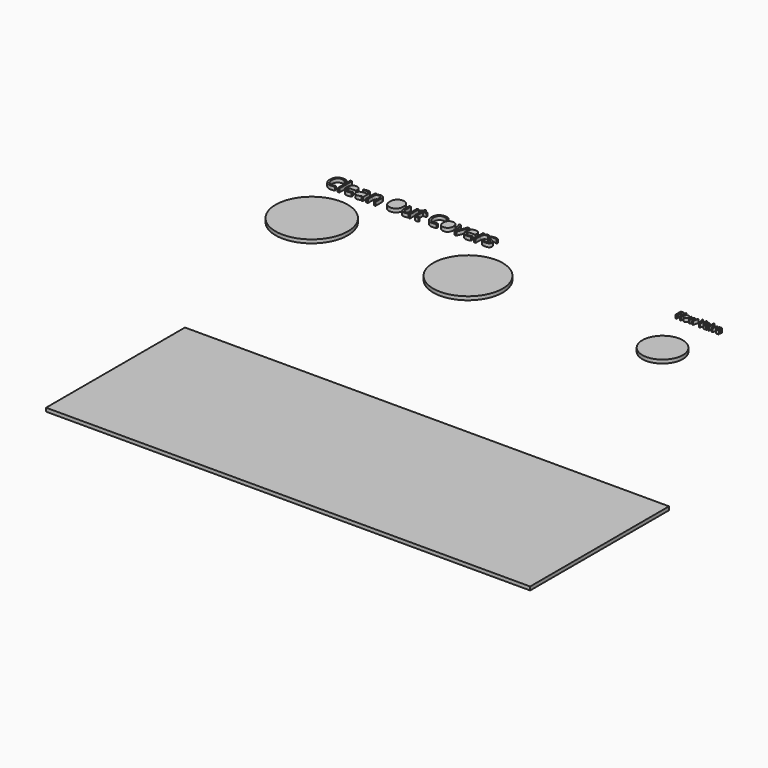
from build123d import *

# Parameters (mm, degrees)
F0_W           = 4170.580181663
F0_H           = 1495.7776816476
F0_W_2         = 38.067660993
F0_H_2         = 356.6917830613
F0_H_3         = 251.2172233158
F0_R           = 311.3295690079
F0_R_2         = 299.2849043025
F0_R_3         = 174.2052882787
F0_TEXT_SIZE   = 179.4427633286
F0_TEXT_SIZE_2 = 469.4278041522
F0_TEXT_SIZE_3 = 78.9547959963
F1_DEPTH       = 30.48


# Not quite as in the source:
# - Text() gives the source's letters only with a copy of the font that has no kerning and outlines rounded to 1/6400 em; it was checked with that copy


with BuildPart() as f1:
    # F0 (on Top) → F1 (new body)
    with BuildSketch(Plane.XY):
        with Locations((453.2191234097, -1260.6751158237)):
            Rectangle(F0_W, F0_H)
        with BuildLine():
            add(Edge.make_bspline(
                [(-404.8579966184, -1421.0070061187), (-364.2965004159, -1466.8495651179), (-364.2965004159, -1547.5324689566)],
                knots=[0, 0, 0, 1, 1, 1], degree=2))
            add(Edge.make_bspline(
                [(-364.2965004159, -1547.5324689566), (-364.2965004159, -1627.995328512), (-405.0046928072, -1674.0946058417)],
                knots=[0, 0, 0, 1, 1, 1], degree=2))
            add(Edge.make_bspline(
                [(-405.0046928072, -1674.0946058417), (-445.7128851985, -1720.1938831713), (-518.1074543701, -1720.1938831713)],
                knots=[0, 0, 0, 1, 1, 1], degree=2))
            add(Edge.make_bspline(
                [(-518.1074543701, -1720.1938831713), (-592.1156816185, -1720.1938831713), (-632.3471113962, -1674.9014348801)],
                knots=[0, 0, 0, 1, 1, 1], degree=2))
            add(Edge.make_bspline(
                [(-632.3471113962, -1674.9014348801), (-672.5785411739, -1629.6089865888), (-672.5785411739, -1547.0923803902)],
                knots=[0, 0, 0, 1, 1, 1], degree=2))
            add(Edge.make_bspline(
                [(-672.5785411739, -1547.0923803902), (-672.5785411739, -1465.2359070412), (-632.2370892546, -1420.2001770803)],
                knots=[0, 0, 0, 1, 1, 1], degree=2))
            add(Edge.make_bspline(
                [(-632.2370892546, -1420.2001770803), (-591.8956373353, -1375.1644471195), (-517.6673658037, -1375.1644471195)],
                knots=[0, 0, 0, 1, 1, 1], degree=2))
            add(Edge.make_bspline(
                [(-517.6673658037, -1375.1644471195), (-445.4194928209, -1375.1644471195), (-404.8579966184, -1421.0070061187)],
                knots=[0, 0, 0, 1, 1, 1], degree=2))
        make_face(mode=Mode.SUBTRACT)
        with Locations((-276.3154611845, -1537.2270616936)):
            Rectangle(F0_W_2, F0_H_2, mode=Mode.SUBTRACT)
        with BuildLine():
            Line((-0.5633002923, -1715.5729532242), (-5.6243188058, -1681.9061778951))
            Line((-5.6243188058, -1681.9061778951), (-7.678065449, -1681.9061778951))
            add(Edge.make_bspline(
                [(-7.678065449, -1681.9061778951), (-34.0100313382, -1720.1938831713), (-86.5272669277, -1720.1938831713)],
                knots=[0, 0, 0, 1, 1, 1], degree=2))
            add(Edge.make_bspline(
                [(-86.5272669277, -1720.1938831713), (-135.8171863637, -1720.1938831713), (-163.2126996216, -1686.4904337951)],
                knots=[0, 0, 0, 1, 1, 1], degree=2))
            add(Edge.make_bspline(
                [(-163.2126996216, -1686.4904337951), (-190.6082128795, -1652.7869844188), (-190.6082128795, -1590.6611484631)],
                knots=[0, 0, 0, 1, 1, 1], degree=2))
            add(Edge.make_bspline(
                [(-190.6082128795, -1590.6611484631), (-190.6082128795, -1528.5353125073), (-163.10267748, -1494.1350562343)],
                knots=[0, 0, 0, 1, 1, 1], degree=2))
            add(Edge.make_bspline(
                [(-163.10267748, -1494.1350562343), (-135.5971420805, -1459.7347999612), (-86.5272669277, -1459.7347999612)],
                knots=[0, 0, 0, 1, 1, 1], degree=2))
            add(Edge.make_bspline(
                [(-86.5272669277, -1459.7347999612), (-35.4036451317, -1459.7347999612), (-8.1181540154, -1496.9222838214)],
                knots=[0, 0, 0, 1, 1, 1], degree=2))
            Line((-8.1181540154, -1496.9222838214), (-5.110882145, -1496.9222838214))
            Line((-5.110882145, -1496.9222838214), (-6.7245402218, -1478.8053045049))
            Line((-6.7245402218, -1478.8053045049), (-7.678065449, -1461.1284137548))
            Line((-7.678065449, -1461.1284137548), (-7.678065449, -1358.8811701629))
            Line((-7.678065449, -1358.8811701629), (30.389595544, -1358.8811701629))
            Line((30.389595544, -1358.8811701629), (30.389595544, -1715.5729532242))
            Line((30.389595544, -1715.5729532242), (-0.5633002923, -1715.5729532242))
        make_face(mode=Mode.SUBTRACT)
        with BuildLine():
            add(Edge.make_bspline(
                [(325.6890235934, -1380.4455099162), (451.2609612041, -1380.4455099162), (451.2609612041, -1478.0718235609)],
                knots=[0, 0, 0, 1, 1, 1], degree=2))
            add(Edge.make_bspline(
                [(451.2609612041, -1478.0718235609), (451.2609612041, -1528.9754010737), (416.5306385063, -1556.3709143316)],
                knots=[0, 0, 0, 1, 1, 1], degree=2))
            add(Edge.make_bspline(
                [(416.5306385063, -1556.3709143316), (381.8003158085, -1583.7664275896), (317.1806446432, -1583.7664275896)],
                knots=[0, 0, 0, 1, 1, 1], degree=2))
            Line((317.1806446432, -1583.7664275896), (277.7193698566, -1583.7664275896))
            Line((277.7193698566, -1583.7664275896), (277.7193698566, -1715.5729532242))
            Line((277.7193698566, -1715.5729532242), (238.7715317309, -1715.5729532242))
            Line((238.7715317309, -1715.5729532242), (238.7715317309, -1380.4455099162))
            Line((238.7715317309, -1380.4455099162), (325.6890235934, -1380.4455099162))
        make_face(mode=Mode.SUBTRACT)
        with BuildLine():
            Line((698.3706912336, -1715.5729532242), (670.1316748901, -1715.5729532242))
            Line((670.1316748901, -1715.5729532242), (662.576821167, -1679.7790831576))
            Line((662.576821167, -1679.7790831576), (660.7431188071, -1679.7790831576))
            add(Edge.make_bspline(
                [(660.7431188071, -1679.7790831576), (641.966006641, -1703.397169554), (623.2989166165, -1711.7955263626)],
                knots=[0, 0, 0, 1, 1, 1], degree=2))
            add(Edge.make_bspline(
                [(623.2989166165, -1711.7955263626), (604.631826592, -1720.1938831713), (576.6128545317, -1720.1938831713)],
                knots=[0, 0, 0, 1, 1, 1], degree=2))
            add(Edge.make_bspline(
                [(576.6128545317, -1720.1938831713), (539.2786744827, -1720.1938831713), (518.0810752014, -1700.9033343444)],
                knots=[0, 0, 0, 1, 1, 1], degree=2))
            add(Edge.make_bspline(
                [(518.0810752014, -1700.9033343444), (496.8834759202, -1681.6127855175), (496.8834759202, -1646.1123078285)],
                knots=[0, 0, 0, 1, 1, 1], degree=2))
            add(Edge.make_bspline(
                [(496.8834759202, -1646.1123078285), (496.8834759202, -1570.050333937), (618.5679645278, -1566.3829292171)],
                knots=[0, 0, 0, 1, 1, 1], degree=2))
            Line((618.5679645278, -1566.3829292171), (661.1832073734, -1564.9893154235))
            Line((661.1832073734, -1564.9893154235), (661.1832073734, -1549.3661713166))
            add(Edge.make_bspline(
                [(661.1832073734, -1549.3661713166), (661.1832073734, -1519.8068892738), (648.4939870425, -1505.7240551493)],
                knots=[0, 0, 0, 1, 1, 1], degree=2))
            add(Edge.make_bspline(
                [(648.4939870425, -1505.7240551493), (635.8047667115, -1491.6412210247), (607.7857946511, -1491.6412210247)],
                knots=[0, 0, 0, 1, 1, 1], degree=2))
            add(Edge.make_bspline(
                [(607.7857946511, -1491.6412210247), (576.3928102485, -1491.6412210247), (536.7848392731, -1510.8584217572)],
                knots=[0, 0, 0, 1, 1, 1], degree=2))
            Line((536.7848392731, -1510.8584217572), (525.0491441693, -1481.7392282809))
            add(Edge.make_bspline(
                [(525.0491441693, -1481.7392282809), (543.6062120522, -1471.6905393482), (565.7206625134, -1465.9693879851)],
                knots=[0, 0, 0, 1, 1, 1], degree=2))
            add(Edge.make_bspline(
                [(565.7206625134, -1465.9693879851), (587.8351129747, -1460.248236622), (610.1329336719, -1460.248236622)],
                knots=[0, 0, 0, 1, 1, 1], degree=2))
            add(Edge.make_bspline(
                [(610.1329336719, -1460.248236622), (655.0219674439, -1460.248236622), (676.6963293388, -1480.1622442513)],
                knots=[0, 0, 0, 1, 1, 1], degree=2))
            add(Edge.make_bspline(
                [(676.6963293388, -1480.1622442513), (698.3706912336, -1500.0762518806), (698.3706912336, -1544.0851085198)],
                knots=[0, 0, 0, 1, 1, 1], degree=2))
            Line((698.3706912336, -1544.0851085198), (698.3706912336, -1715.5729532242))
        make_face(mode=Mode.SUBTRACT)
        with BuildLine():
            add(Edge.make_bspline(
                [(828.2701664139, -1676.5884410512), (839.0523362905, -1688.7275506742), (857.8294484566, -1688.7275506742)],
                knots=[0, 0, 0, 1, 1, 1], degree=2))
            add(Edge.make_bspline(
                [(857.8294484566, -1688.7275506742), (867.9514854836, -1688.7275506742), (877.3400415666, -1687.2605887863)],
                knots=[0, 0, 0, 1, 1, 1], degree=2))
            add(Edge.make_bspline(
                [(877.3400415666, -1687.2605887863), (886.7285976497, -1685.7936268983), (892.2297047296, -1684.1799688215)],
                knots=[0, 0, 0, 1, 1, 1], degree=2))
            Line((892.2297047296, -1684.1799688215), (892.2297047296, -1713.2991622978))
            add(Edge.make_bspline(
                [(892.2297047296, -1713.2991622978), (886.0684648001, -1716.2330860738), (874.0393773187, -1718.2134846225)],
                knots=[0, 0, 0, 1, 1, 1], degree=2))
            add(Edge.make_bspline(
                [(874.0393773187, -1718.2134846225), (862.0102898373, -1720.1938831713), (852.3283413767, -1720.1938831713)],
                knots=[0, 0, 0, 1, 1, 1], degree=2))
            add(Edge.make_bspline(
                [(852.3283413767, -1720.1938831713), (779.4936836387, -1720.1938831713), (779.4936836387, -1643.3984283358)],
                knots=[0, 0, 0, 1, 1, 1], degree=2))
            Line((779.4936836387, -1643.3984283358), (779.4936836387, -1493.9150119511))
            Line((779.4936836387, -1493.9150119511), (743.4797692889, -1493.9150119511))
            Line((743.4797692889, -1493.9150119511), (743.4797692889, -1475.5779883514))
            Line((743.4797692889, -1475.5779883514), (779.4936836387, -1459.7347999612))
            Line((779.4936836387, -1459.7347999612), (795.4835682176, -1406.1173429557))
            Line((795.4835682176, -1406.1173429557), (817.4879965372, -1406.1173429557))
            Line((817.4879965372, -1406.1173429557), (817.4879965372, -1464.3557299084))
            Line((817.4879965372, -1464.3557299084), (890.3960023696, -1464.3557299084))
            Line((890.3960023696, -1464.3557299084), (890.3960023696, -1493.9150119511))
            Line((890.3960023696, -1493.9150119511), (817.4879965372, -1493.9150119511))
            Line((817.4879965372, -1493.9150119511), (817.4879965372, -1641.784770259))
            add(Edge.make_bspline(
                [(817.4879965372, -1641.784770259), (817.4879965372, -1664.4493314282), (828.2701664139, -1676.5884410512)],
                knots=[0, 0, 0, 1, 1, 1], degree=2))
        make_face(mode=Mode.SUBTRACT)
        with Locations((961.4336317948, -1589.9643415663)):
            Rectangle(F0_W_2, F0_H_3, mode=Mode.SUBTRACT)
        with BuildLine():
            add(Edge.make_bspline(
                [(1246.9044151949, -1494.8318631311), (1277.9673331728, -1529.9289263009), (1277.9673331728, -1589.7076232359)],
                knots=[0, 0, 0, 1, 1, 1], degree=2))
            add(Edge.make_bspline(
                [(1277.9673331728, -1589.7076232359), (1277.9673331728, -1651.1733263421), (1247.0511113837, -1685.6836047567)],
                knots=[0, 0, 0, 1, 1, 1], degree=2))
            add(Edge.make_bspline(
                [(1247.0511113837, -1685.6836047567), (1216.1348895946, -1720.1938831713), (1161.5639073619, -1720.1938831713)],
                knots=[0, 0, 0, 1, 1, 1], degree=2))
            add(Edge.make_bspline(
                [(1161.5639073619, -1720.1938831713), (1127.8237839385, -1720.1938831713), (1101.7118623325, -1704.3506947812)],
                knots=[0, 0, 0, 1, 1, 1], degree=2))
            add(Edge.make_bspline(
                [(1101.7118623325, -1704.3506947812), (1075.5999407265, -1688.507506391), (1061.3704104132, -1658.9482243483)],
                knots=[0, 0, 0, 1, 1, 1], degree=2))
            add(Edge.make_bspline(
                [(1061.3704104132, -1658.9482243483), (1047.1408800998, -1629.3889423056), (1047.1408800998, -1589.7076232359)],
                knots=[0, 0, 0, 1, 1, 1], degree=2))
            add(Edge.make_bspline(
                [(1047.1408800998, -1589.7076232359), (1047.1408800998, -1528.3152682241), (1077.8737316529, -1494.0250340927)],
                knots=[0, 0, 0, 1, 1, 1], degree=2))
            add(Edge.make_bspline(
                [(1077.8737316529, -1494.0250340927), (1108.606583206, -1459.7347999612), (1163.1775654387, -1459.7347999612)],
                knots=[0, 0, 0, 1, 1, 1], degree=2))
            add(Edge.make_bspline(
                [(1163.1775654387, -1459.7347999612), (1215.841497217, -1459.7347999612), (1246.9044151949, -1494.8318631311)],
                knots=[0, 0, 0, 1, 1, 1], degree=2))
        make_face(mode=Mode.SUBTRACT)
        with BuildLine():
            add(Edge.make_bspline(
                [(945.5904434047, -1415.4325509444), (939.1724851448, -1409.1246148261), (939.1724851448, -1396.2886983063)],
                knots=[0, 0, 0, 1, 1, 1], degree=2))
            add(Edge.make_bspline(
                [(939.1724851448, -1396.2886983063), (939.1724851448, -1383.2327375033), (945.5904434047, -1377.1448456682)],
                knots=[0, 0, 0, 1, 1, 1], degree=2))
            add(Edge.make_bspline(
                [(945.5904434047, -1377.1448456682), (952.0084016646, -1371.0569538331), (961.6903501252, -1371.0569538331)],
                knots=[0, 0, 0, 1, 1, 1], degree=2))
            add(Edge.make_bspline(
                [(961.6903501252, -1371.0569538331), (970.8588619251, -1371.0569538331), (977.4968644682, -1377.2548678098)],
                knots=[0, 0, 0, 1, 1, 1], degree=2))
            add(Edge.make_bspline(
                [(977.4968644682, -1377.2548678098), (984.1348670113, -1383.4527817865), (984.1348670113, -1396.2886983063)],
                knots=[0, 0, 0, 1, 1, 1], degree=2))
            add(Edge.make_bspline(
                [(984.1348670113, -1396.2886983063), (984.1348670113, -1409.1246148261), (977.4968644682, -1415.4325509444)],
                knots=[0, 0, 0, 1, 1, 1], degree=2))
            add(Edge.make_bspline(
                [(977.4968644682, -1415.4325509444), (970.8588619251, -1421.7404870627), (961.6903501252, -1421.7404870627)],
                knots=[0, 0, 0, 1, 1, 1], degree=2))
            add(Edge.make_bspline(
                [(961.6903501252, -1421.7404870627), (952.0084016646, -1421.7404870627), (945.5904434047, -1415.4325509444)],
                knots=[0, 0, 0, 1, 1, 1], degree=2))
        make_face(mode=Mode.SUBTRACT)
        with Locations((-1962.2709674218, 1265.2137250001)):
            Circle(F0_R)
        with Locations((-616.0709674218, 1265.2137250001)):
            Circle(F0_R_2)
        with Locations((1060.3290325782, 1265.2137250001)):
            Circle(F0_R_3)
        with BuildLine():
            add(Edge.make_bspline(
                [(-602.3477407871, -1445.2118772703), (-631.3569121218, -1480.4189625817), (-631.3569121218, -1547.5324689566)],
                knots=[0, 0, 0, 1, 1, 1], degree=2))
            add(Edge.make_bspline(
                [(-631.3569121218, -1547.5324689566), (-631.3569121218, -1615.5995005586), (-602.3477407871, -1650.8065858701)],
                knots=[0, 0, 0, 1, 1, 1], degree=2))
            add(Edge.make_bspline(
                [(-602.3477407871, -1650.8065858701), (-573.3385694524, -1686.0136711815), (-518.1074543701, -1686.0136711815)],
                knots=[0, 0, 0, 1, 1, 1], degree=2))
            add(Edge.make_bspline(
                [(-518.1074543701, -1686.0136711815), (-462.4362507214, -1686.0136711815), (-434.0138641419, -1650.9532820589)],
                knots=[0, 0, 0, 1, 1, 1], degree=2))
            add(Edge.make_bspline(
                [(-434.0138641419, -1650.9532820589), (-405.5914775624, -1615.8928929362), (-405.5914775624, -1547.5324689566)],
                knots=[0, 0, 0, 1, 1, 1], degree=2))
            add(Edge.make_bspline(
                [(-405.5914775624, -1547.5324689566), (-405.5914775624, -1479.9055259209), (-433.9038420003, -1444.9551589399)],
                knots=[0, 0, 0, 1, 1, 1], degree=2))
            add(Edge.make_bspline(
                [(-433.9038420003, -1444.9551589399), (-462.2162064382, -1410.0047919589), (-517.6673658037, -1410.0047919589)],
                knots=[0, 0, 0, 1, 1, 1], degree=2))
            add(Edge.make_bspline(
                [(-517.6673658037, -1410.0047919589), (-573.3385694524, -1410.0047919589), (-602.3477407871, -1445.2118772703)],
                knots=[0, 0, 0, 1, 1, 1], degree=2))
        make_face()
        with BuildLine():
            add(Edge.make_bspline(
                [(1105.6359853828, -1516.6162471675), (1086.6021548863, -1541.1511847439), (1086.6021548863, -1589.7076232359)],
                knots=[0, 0, 0, 1, 1, 1], degree=2))
            add(Edge.make_bspline(
                [(1086.6021548863, -1589.7076232359), (1086.6021548863, -1637.8973212559), (1105.856029666, -1663.0923916819)],
                knots=[0, 0, 0, 1, 1, 1], degree=2))
            add(Edge.make_bspline(
                [(1105.856029666, -1663.0923916819), (1125.1099044457, -1688.2874621078), (1162.4440844947, -1688.2874621078)],
                knots=[0, 0, 0, 1, 1, 1], degree=2))
            add(Edge.make_bspline(
                [(1162.4440844947, -1688.2874621078), (1199.8516126381, -1688.2874621078), (1219.2155095593, -1663.2024138235)],
                knots=[0, 0, 0, 1, 1, 1], degree=2))
            add(Edge.make_bspline(
                [(1219.2155095593, -1663.2024138235), (1238.5794064806, -1638.1173655391), (1238.5794064806, -1589.7076232359)],
                knots=[0, 0, 0, 1, 1, 1], degree=2))
            add(Edge.make_bspline(
                [(1238.5794064806, -1589.7076232359), (1238.5794064806, -1541.8113175935), (1219.2155095593, -1516.9463135923)],
                knots=[0, 0, 0, 1, 1, 1], degree=2))
            add(Edge.make_bspline(
                [(1219.2155095593, -1516.9463135923), (1199.8516126381, -1492.0813095911), (1162.0039959283, -1492.0813095911)],
                knots=[0, 0, 0, 1, 1, 1], degree=2))
            add(Edge.make_bspline(
                [(1162.0039959283, -1492.0813095911), (1124.6698158793, -1492.0813095911), (1105.6359853828, -1516.6162471675)],
                knots=[0, 0, 0, 1, 1, 1], degree=2))
        make_face()
        with BuildLine():
            add(Edge.make_bspline(
                [(-133.5067213901, -1663.7525245314), (-115.8665046872, -1688.2874621078), (-81.6862926974, -1688.2874621078)],
                knots=[0, 0, 0, 1, 1, 1], degree=2))
            add(Edge.make_bspline(
                [(-81.6862926974, -1688.2874621078), (-42.7384545716, -1688.2874621078), (-25.2082600103, -1667.0898628266)],
                knots=[0, 0, 0, 1, 1, 1], degree=2))
            add(Edge.make_bspline(
                [(-25.2082600103, -1667.0898628266), (-7.678065449, -1645.8922635453), (-7.678065449, -1598.6560907525)],
                knots=[0, 0, 0, 1, 1, 1], degree=2))
            Line((-7.678065449, -1598.6560907525), (-7.678065449, -1590.6611484631))
            add(Edge.make_bspline(
                [(-7.678065449, -1590.6611484631), (-7.678065449, -1537.2637357408), (-25.4283042935, -1514.4524783827)],
                knots=[0, 0, 0, 1, 1, 1], degree=2))
            add(Edge.make_bspline(
                [(-25.4283042935, -1514.4524783827), (-43.178543138, -1491.6412210247), (-82.1263812638, -1491.6412210247)],
                knots=[0, 0, 0, 1, 1, 1], degree=2))
            add(Edge.make_bspline(
                [(-82.1263812638, -1491.6412210247), (-115.646460404, -1491.6412210247), (-133.3966992485, -1517.6431204891)],
                knots=[0, 0, 0, 1, 1, 1], degree=2))
            add(Edge.make_bspline(
                [(-133.3966992485, -1517.6431204891), (-151.146938093, -1543.6450199534), (-151.146938093, -1591.1012370295)],
                knots=[0, 0, 0, 1, 1, 1], degree=2))
            add(Edge.make_bspline(
                [(-151.146938093, -1591.1012370295), (-151.146938093, -1639.2175869551), (-133.5067213901, -1663.7525245314)],
                knots=[0, 0, 0, 1, 1, 1], degree=2))
        make_face()
        with BuildLine():
            Line((277.7193698566, -1414.1856333396), (277.7193698566, -1550.3196965437))
            Line((277.7193698566, -1550.3196965437), (312.8531070737, -1550.3196965437))
            add(Edge.make_bspline(
                [(312.8531070737, -1550.3196965437), (364.6368617192, -1550.3196965437), (387.778185502, -1533.5963310208)],
                knots=[0, 0, 0, 1, 1, 1], degree=2))
            add(Edge.make_bspline(
                [(387.778185502, -1533.5963310208), (410.9195092848, -1516.8729654979), (410.9195092848, -1479.9055259209)],
                knots=[0, 0, 0, 1, 1, 1], degree=2))
            add(Edge.make_bspline(
                [(410.9195092848, -1479.9055259209), (410.9195092848, -1446.6788391583), (389.1351252484, -1430.4322362489)],
                knots=[0, 0, 0, 1, 1, 1], degree=2))
            add(Edge.make_bspline(
                [(389.1351252484, -1430.4322362489), (367.3507412119, -1414.1856333396), (321.2881379295, -1414.1856333396)],
                knots=[0, 0, 0, 1, 1, 1], degree=2))
            Line((321.2881379295, -1414.1856333396), (277.7193698566, -1414.1856333396))
        make_face()
        with BuildLine():
            add(Edge.make_bspline(
                [(549.2540153209, -1677.9820548448), (561.7231913687, -1688.7275506742), (584.1677082547, -1688.7275506742)],
                knots=[0, 0, 0, 1, 1, 1], degree=2))
            add(Edge.make_bspline(
                [(584.1677082547, -1688.7275506742), (619.7415340381, -1688.7275506742), (640.0222821394, -1669.2536316114)],
                knots=[0, 0, 0, 1, 1, 1], degree=2))
            add(Edge.make_bspline(
                [(640.0222821394, -1669.2536316114), (660.3030302407, -1649.7797125485), (660.3030302407, -1614.7193234259)],
                knots=[0, 0, 0, 1, 1, 1], degree=2))
            Line((660.3030302407, -1614.7193234259), (660.3030302407, -1592.0547622566))
            Line((660.3030302407, -1592.0547622566), (622.2353692477, -1593.595072239))
            add(Edge.make_bspline(
                [(622.2353692477, -1593.595072239), (576.8328988149, -1595.2087303158), (556.808869044, -1607.7145804108)],
                knots=[0, 0, 0, 1, 1, 1], degree=2))
            add(Edge.make_bspline(
                [(556.808869044, -1607.7145804108), (536.7848392731, -1620.2204305058), (536.7848392731, -1646.5523963949)],
                knots=[0, 0, 0, 1, 1, 1], degree=2))
            add(Edge.make_bspline(
                [(536.7848392731, -1646.5523963949), (536.7848392731, -1667.2365590154), (549.2540153209, -1677.9820548448)],
                knots=[0, 0, 0, 1, 1, 1], degree=2))
        make_face()
        with BuildLine():
            add(Edge.make_bspline(
                [(-1675.3814967815, 1820.7862759009), (-1686.4704987966, 1807.3280686513), (-1686.4704987966, 1781.6733610816)],
                knots=[0, 0, 0, 1, 1, 1], degree=2))
            add(Edge.make_bspline(
                [(-1686.4704987966, 1781.6733610816), (-1686.4704987966, 1755.654160399), (-1675.3814967815, 1742.1959531493)],
                knots=[0, 0, 0, 1, 1, 1], degree=2))
            add(Edge.make_bspline(
                [(-1675.3814967815, 1742.1959531493), (-1664.2924947664, 1728.7377458997), (-1643.1799321435, 1728.7377458997)],
                knots=[0, 0, 0, 1, 1, 1], degree=2))
            add(Edge.make_bspline(
                [(-1643.1799321435, 1728.7377458997), (-1621.89914193, 1728.7377458997), (-1611.0344433691, 1742.1398772858)],
                knots=[0, 0, 0, 1, 1, 1], degree=2))
            add(Edge.make_bspline(
                [(-1611.0344433691, 1742.1398772858), (-1600.1697448082, 1755.5420086719), (-1600.1697448082, 1781.6733610816)],
                knots=[0, 0, 0, 1, 1, 1], degree=2))
            add(Edge.make_bspline(
                [(-1600.1697448082, 1781.6733610816), (-1600.1697448082, 1807.5243341736), (-1610.9923864715, 1820.8844086621)],
                knots=[0, 0, 0, 1, 1, 1], degree=2))
            add(Edge.make_bspline(
                [(-1610.9923864715, 1820.8844086621), (-1621.8150281347, 1834.2444831505), (-1643.0117045529, 1834.2444831505)],
                knots=[0, 0, 0, 1, 1, 1], degree=2))
            add(Edge.make_bspline(
                [(-1643.0117045529, 1834.2444831505), (-1664.2924947664, 1834.2444831505), (-1675.3814967815, 1820.7862759009)],
                knots=[0, 0, 0, 1, 1, 1], degree=2))
        make_face()
        with BuildLine():
            add(Edge.make_bspline(
                [(-1207.7087948564, 1793.4913493227), (-1214.9846381508, 1784.1126611456), (-1214.9846381508, 1765.5515503138)],
                knots=[0, 0, 0, 1, 1, 1], degree=2))
            add(Edge.make_bspline(
                [(-1214.9846381508, 1765.5515503138), (-1214.9846381508, 1747.1306291409), (-1207.6246810611, 1737.4995995779)],
                knots=[0, 0, 0, 1, 1, 1], degree=2))
            add(Edge.make_bspline(
                [(-1207.6246810611, 1737.4995995779), (-1200.2647239715, 1727.8685700148), (-1185.9934167005, 1727.8685700148)],
                knots=[0, 0, 0, 1, 1, 1], degree=2))
            add(Edge.make_bspline(
                [(-1185.9934167005, 1727.8685700148), (-1171.6940714978, 1727.8685700148), (-1164.2920575105, 1737.4575426802)],
                knots=[0, 0, 0, 1, 1, 1], degree=2))
            add(Edge.make_bspline(
                [(-1164.2920575105, 1737.4575426802), (-1156.8900435232, 1747.0465153456), (-1156.8900435232, 1765.5515503138)],
                knots=[0, 0, 0, 1, 1, 1], degree=2))
            add(Edge.make_bspline(
                [(-1156.8900435232, 1765.5515503138), (-1156.8900435232, 1783.8603197597), (-1164.2920575105, 1793.3651786298)],
                knots=[0, 0, 0, 1, 1, 1], degree=2))
            add(Edge.make_bspline(
                [(-1164.2920575105, 1793.3651786298), (-1171.6940714978, 1802.8700374998), (-1186.1616442911, 1802.8700374998)],
                knots=[0, 0, 0, 1, 1, 1], degree=2))
            add(Edge.make_bspline(
                [(-1186.1616442911, 1802.8700374998), (-1200.4329515621, 1802.8700374998), (-1207.7087948564, 1793.4913493227)],
                knots=[0, 0, 0, 1, 1, 1], degree=2))
        make_face()
        with Locations((-2229.0325164795, 1717.4384593964)):
            Text('Clean Out Covers', F0_TEXT_SIZE, font='Open Sans', text_align=(TextAlign.LEFT, TextAlign.BOTTOM))
        with Locations((-701.2576460838, -1715.5729532242)):
            Text('Old Patio', F0_TEXT_SIZE_2, font='Open Sans', text_align=(TextAlign.LEFT, TextAlign.BOTTOM))
        with BuildLine():
            add(Edge.make_bspline(
                [(-1941.4754882455, 1731.8078994285), (-1936.7090398446, 1727.7003424242), (-1928.1294327229, 1727.7003424242)],
                knots=[0, 0, 0, 1, 1, 1], degree=2))
            add(Edge.make_bspline(
                [(-1928.1294327229, 1727.7003424242), (-1914.5310358144, 1727.7003424242), (-1906.77854768, 1735.1444133092)],
                knots=[0, 0, 0, 1, 1, 1], degree=2))
            add(Edge.make_bspline(
                [(-1906.77854768, 1735.1444133092), (-1899.0260595456, 1742.5884841941), (-1899.0260595456, 1755.9906155802)],
                knots=[0, 0, 0, 1, 1, 1], degree=2))
            Line((-1899.0260595456, 1755.9906155802), (-1899.0260595456, 1764.6543364972))
            Line((-1899.0260595456, 1764.6543364972), (-1913.5777461343, 1764.06553993))
            add(Edge.make_bspline(
                [(-1913.5777461343, 1764.06553993), (-1930.9332258999, 1763.4487054311), (-1938.5875812732, 1758.6682380643)],
                knots=[0, 0, 0, 1, 1, 1], degree=2))
            add(Edge.make_bspline(
                [(-1938.5875812732, 1758.6682380643), (-1946.2419366464, 1753.8877706975), (-1946.2419366464, 1743.822153192)],
                knots=[0, 0, 0, 1, 1, 1], degree=2))
            add(Edge.make_bspline(
                [(-1946.2419366464, 1743.822153192), (-1946.2419366464, 1735.9154564328), (-1941.4754882455, 1731.8078994285)],
                knots=[0, 0, 0, 1, 1, 1], degree=2))
        make_face()
        with BuildLine():
            add(Edge.make_bspline(
                [(-2000.8458087686, 1795.7203648984), (-2006.9720968604, 1803.0382650904), (-2018.3835350908, 1803.0382650904)],
                knots=[0, 0, 0, 1, 1, 1], degree=2))
            add(Edge.make_bspline(
                [(-2018.3835350908, 1803.0382650904), (-2029.9351629801, 1803.0382650904), (-2036.8184752297, 1795.5100804102)],
                knots=[0, 0, 0, 1, 1, 1], degree=2))
            add(Edge.make_bspline(
                [(-2036.8184752297, 1795.5100804102), (-2043.7017874792, 1787.9818957299), (-2044.9354564771, 1774.6638781391)],
                knots=[0, 0, 0, 1, 1, 1], degree=2))
            Line((-2044.9354564771, 1774.6638781391), (-1994.7195206769, 1774.6638781391))
            add(Edge.make_bspline(
                [(-1994.7195206769, 1774.6638781391), (-1994.7195206769, 1788.4024647065), (-2000.8458087686, 1795.7203648984)],
                knots=[0, 0, 0, 1, 1, 1], degree=2))
        make_face()
        with BuildLine():
            add(Edge.make_bspline(
                [(-972.274281783, 1795.7203648984), (-978.4005698748, 1803.0382650904), (-989.8120081052, 1803.0382650904)],
                knots=[0, 0, 0, 1, 1, 1], degree=2))
            add(Edge.make_bspline(
                [(-989.8120081052, 1803.0382650904), (-1001.3636359945, 1803.0382650904), (-1008.2469482441, 1795.5100804102)],
                knots=[0, 0, 0, 1, 1, 1], degree=2))
            add(Edge.make_bspline(
                [(-1008.2469482441, 1795.5100804102), (-1015.1302604936, 1787.9818957299), (-1016.3639294915, 1774.6638781391)],
                knots=[0, 0, 0, 1, 1, 1], degree=2))
            Line((-1016.3639294915, 1774.6638781391), (-966.1479936913, 1774.6638781391))
            add(Edge.make_bspline(
                [(-966.1479936913, 1774.6638781391), (-966.1479936913, 1788.4024647065), (-972.274281783, 1795.7203648984)],
                knots=[0, 0, 0, 1, 1, 1], degree=2))
        make_face()
        with BuildLine():
            add(Edge.make_bspline(
                [(895.0481486584, 1730.2299972701), (891.8467784145, 1726.1033755106), (891.8467784145, 1717.9364887998)],
                knots=[0, 0, 0, 1, 1, 1], degree=2))
            add(Edge.make_bspline(
                [(891.8467784145, 1717.9364887998), (891.8467784145, 1709.8312855233), (895.0851587191, 1705.5936335819)],
                knots=[0, 0, 0, 1, 1, 1], degree=2))
            add(Edge.make_bspline(
                [(895.0851587191, 1705.5936335819), (898.3235390236, 1701.3559816405), (904.6029126427, 1701.3559816405)],
                knots=[0, 0, 0, 1, 1, 1], degree=2))
            add(Edge.make_bspline(
                [(904.6029126427, 1701.3559816405), (910.8946229486, 1701.3559816405), (914.1515082835, 1705.5751285516)],
                knots=[0, 0, 0, 1, 1, 1], degree=2))
            add(Edge.make_bspline(
                [(914.1515082835, 1705.5751285516), (917.4083936183, 1709.7942754626), (917.4083936183, 1717.9364887998)],
                knots=[0, 0, 0, 1, 1, 1], degree=2))
            add(Edge.make_bspline(
                [(917.4083936183, 1717.9364887998), (917.4083936183, 1725.9923453288), (914.1515082835, 1730.1744821792)],
                knots=[0, 0, 0, 1, 1, 1], degree=2))
            add(Edge.make_bspline(
                [(914.1515082835, 1730.1744821792), (910.8946229486, 1734.3566190296), (904.5288925214, 1734.3566190296)],
                knots=[0, 0, 0, 1, 1, 1], degree=2))
            add(Edge.make_bspline(
                [(904.5288925214, 1734.3566190296), (898.2495189024, 1734.3566190296), (895.0481486584, 1730.2299972701)],
                knots=[0, 0, 0, 1, 1, 1], degree=2))
        make_face()
        with Locations((820.0595974922, 1696.7667341232)):
            Text('Flow Valve', F0_TEXT_SIZE_3, font='Open Sans', text_align=(TextAlign.LEFT, TextAlign.BOTTOM))
        with BuildLine():
            add(Edge.make_bspline(
                [(1069.8281599519, 1703.0892861464), (1071.9253967206, 1701.2819615193), (1075.7004229041, 1701.2819615193)],
                knots=[0, 0, 0, 1, 1, 1], degree=2))
            add(Edge.make_bspline(
                [(1075.7004229041, 1701.2819615193), (1081.6837160382, 1701.2819615193), (1085.094809959, 1704.5573518844)],
                knots=[0, 0, 0, 1, 1, 1], degree=2))
            add(Edge.make_bspline(
                [(1085.094809959, 1704.5573518844), (1088.5059038798, 1707.8327422496), (1088.5059038798, 1713.7296785756)],
                knots=[0, 0, 0, 1, 1, 1], degree=2))
            Line((1088.5059038798, 1713.7296785756), (1088.5059038798, 1717.5417148198))
            Line((1088.5059038798, 1717.5417148198), (1082.103163392, 1717.2826443954))
            add(Edge.make_bspline(
                [(1082.103163392, 1717.2826443954), (1074.4667542167, 1717.0112372842), (1071.0988387, 1714.9078321721)],
                knots=[0, 0, 0, 1, 1, 1], degree=2))
            add(Edge.make_bspline(
                [(1071.0988387, 1714.9078321721), (1067.7309231833, 1712.80442706), (1067.7309231833, 1708.3755564721)],
                knots=[0, 0, 0, 1, 1, 1], degree=2))
            add(Edge.make_bspline(
                [(1067.7309231833, 1708.3755564721), (1067.7309231833, 1704.8966107735), (1069.8281599519, 1703.0892861464)],
                knots=[0, 0, 0, 1, 1, 1], degree=2))
        make_face()
        with BuildLine():
            add(Edge.make_bspline(
                [(1191.4370508166, 1731.2107638766), (1188.7414847345, 1734.4306391509), (1183.7204531766, 1734.4306391509)],
                knots=[0, 0, 0, 1, 1, 1], degree=2))
            add(Edge.make_bspline(
                [(1183.7204531766, 1734.4306391509), (1178.6377381844, 1734.4306391509), (1175.6090815567, 1731.1182387251)],
                knots=[0, 0, 0, 1, 1, 1], degree=2))
            add(Edge.make_bspline(
                [(1175.6090815567, 1731.1182387251), (1172.580424929, 1727.8058382993), (1172.0376107066, 1721.9459120339)],
                knots=[0, 0, 0, 1, 1, 1], degree=2))
            Line((1172.0376107066, 1721.9459120339), (1194.1326168987, 1721.9459120339))
            add(Edge.make_bspline(
                [(1194.1326168987, 1721.9459120339), (1194.1326168987, 1727.9908886024), (1191.4370508166, 1731.2107638766)],
                knots=[0, 0, 0, 1, 1, 1], degree=2))
        make_face()
    extrude(amount=F1_DEPTH)


solid = f1.part
